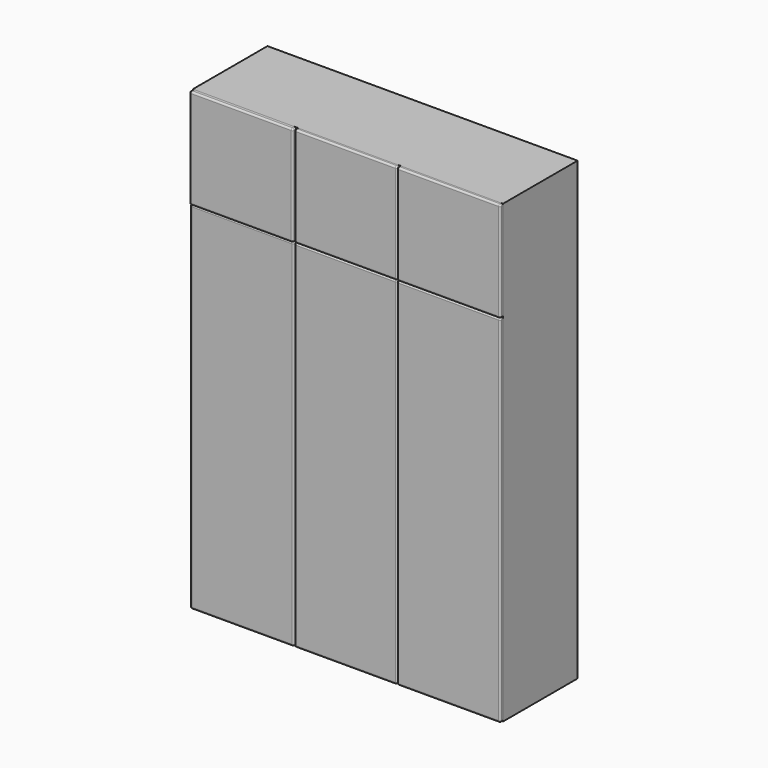
from build123d import *

# Parameters (mm, degrees)
F0_W      = 580
F0_H      = 280
F0_H_2    = 285
F0_H_3    = 175
F0_H_4    = 275
F0_H_5    = 560
F1_DEPTH  = 550
F0_W_2    = 590
F0_H_6    = 20
F5_W      = 610
F5_H      = 2100
F6_DEPTH  = 20
F7_R      = 10
F5_W_2    = 605
F8_DEPTH  = 20
F9_R      = 10
F10_DEPTH = 20
F11_R     = 10
F5_H_2    = 590
F12_DEPTH = 20
F13_R     = 10
F14_DEPTH = 20
F15_R     = 10
F16_DEPTH = 25
F17_R     = 10


# Not quite as in the source:
# - a feature names something its author has since deleted; it is built from what else it names
# - the program builds the solid bodies; features that only make, move or delete a surface that nothing else refers to are left out


with BuildPart() as f1:
    # F0 (on Front) → F1 (new body)
    with BuildSketch(Plane.XZ):
        Polygon((895, -1345), (915, -1345), (915, 1345), (-915, 1345), (-915, -1345), (-895, -1345), (-895, -755), (-315, -755), (-315, -1345), (-295, -1345), (-295, -395), (-295, -375), (-295, 625), (-295, 645), (-295, 745), (295, 745), (295, 645), (295, 625), (295, -375), (295, -395), (295, -1345), (315, -1345), (315, -1320), (315, -1140), (895, -1140), (895, -1320), align=None)
        with Locations((-605, -595)):
            Rectangle(F0_W, F0_H, mode=Mode.SUBTRACT)
        with Locations((-605, -292.5)):
            Rectangle(F0_W, F0_H_2, mode=Mode.SUBTRACT)
        with Locations((605, -1032.5)):
            Rectangle(F0_W, F0_H_3, mode=Mode.SUBTRACT)
        Polygon((315, 745), (895, 745), (895, 645), (895, 625), (895, -925), (315, -925), (315, 625), (315, 645), align=None, mode=Mode.SUBTRACT)
        with Locations((-605, 10)):
            Rectangle(F0_W, F0_H, mode=Mode.SUBTRACT)
        with Locations((-605, 310)):
            Rectangle(F0_W, F0_H, mode=Mode.SUBTRACT)
        with Locations((-605, 607.5)):
            Rectangle(F0_W, F0_H_4, mode=Mode.SUBTRACT)
        with Locations((-605, 1045)):
            Rectangle(F0_W, F0_H_5, mode=Mode.SUBTRACT)
        Polygon((-295, 1325), (895, 1325), (895, 765), (315, 765), (295, 765), (-295, 765), align=None, mode=Mode.SUBTRACT)
    extrude(amount=-F1_DEPTH)


with BuildPart() as f2:
    # F0 (on Front) → F2 (revolve)
    with BuildSketch(Plane.XZ):
        with Locations((0, 635)):
            Rectangle(F0_W_2, F0_H_6)
    revolve(axis=Axis((0, 0, 625), (-1, 0, 0)))


with BuildPart() as f2b:
    # F0 (on Front) → F2, piece 2 (revolve)
    with BuildSketch(Plane.XZ):
        with Locations((605, 635)):
            Rectangle(F0_W, F0_H_6)
    revolve(axis=Axis((0, 0, 625), (-1, 0, 0)))


with BuildPart() as f2_1:
    # F4: moved
    add(f2.part.moved(Location((0, 250, 0))))


with BuildPart() as f2b_1:
    # F4: moved
    add(f2b.part.moved(Location((0, 250, 0))))


with BuildPart() as f6:
    # F5 (on Front) → F6 (new body)
    with BuildSketch(Plane.XZ):
        with Locations((-610, -295)):
            Rectangle(F5_W, F5_H)
    extrude(amount=F6_DEPTH)

    # F7
    f7_edges = [f6.edges().sort_by_distance(p)[0] for p in [
        (-305, -10, 755),
        (-915, -10, 755),
        (-915, -10, -1345),
        (-305, -10, -1345),
        (-610, -20, -1345),
        (-305, -20, -295),
        (-610, -20, 755),
        (-915, -20, -295),
    ]]
    fillet(f7_edges, radius=F7_R)


with BuildPart() as f8:
    # F5 (on Front) → F8 (new body)
    with BuildSketch(Plane.XZ):
        with Locations((2.5, -295)):
            Rectangle(F5_W_2, F5_H)
    extrude(amount=F8_DEPTH)

    # F9
    f9_edges = [f8.edges().sort_by_distance(p)[0] for p in [
        (2.5, -20, -1345),
        (305, -20, -295),
        (2.5, -20, 755),
        (-300, -20, -295),
        (305, -10, 755),
        (-300, -10, 755),
        (305, -10, -1345),
        (-300, -10, -1345),
    ]]
    fillet(f9_edges, radius=F9_R)


with BuildPart() as f10:
    # F5 (on Front) → F10 (new body)
    with BuildSketch(Plane.XZ):
        with Locations((610, -295)):
            Rectangle(F5_W, F5_H)
    extrude(amount=F10_DEPTH)

    # F11
    f11_edges = [f10.edges().sort_by_distance(p)[0] for p in [
        (610, -20, -1345),
        (915, -20, -295),
        (610, -20, 755),
        (305, -20, -295),
        (915, -10, 755),
        (305, -10, 755),
        (305, -10, -1345),
        (915, -10, -1345),
    ]]
    fillet(f11_edges, radius=F11_R)


with BuildPart() as f12:
    # F5 (on Front) → F12 (new body)
    with BuildSketch(Plane.XZ):
        with Locations((610, 1050)):
            Rectangle(F5_W, F5_H_2)
    extrude(amount=F12_DEPTH)

    # F13
    f13_edges = [f12.edges().sort_by_distance(p)[0] for p in [
        (610, -20, 755),
        (915, -20, 1050),
        (610, -20, 1345),
        (305, -20, 1050),
        (915, -10, 1345),
        (915, -10, 755),
        (305, -10, 1345),
        (305, -10, 755),
    ]]
    fillet(f13_edges, radius=F13_R)


with BuildPart() as f14:
    # F5 (on Front) → F14 (new body)
    with BuildSketch(Plane.XZ):
        with Locations((2.5, 1050)):
            Rectangle(F5_W_2, F5_H_2)
    extrude(amount=F14_DEPTH)

    # F15
    f15_edges = [f14.edges().sort_by_distance(p)[0] for p in [
        (2.5, -20, 755),
        (305, -20, 1050),
        (2.5, -20, 1345),
        (-300, -20, 1050),
        (-300, -10, 1345),
        (305, -10, 1345),
        (305, -10, 755),
        (-300, -10, 755),
    ]]
    fillet(f15_edges, radius=F15_R)


with BuildPart() as f16:
    # F5 (on Front) → F16 (new body)
    with BuildSketch(Plane.XZ):
        with Locations((-610, 1050)):
            Rectangle(F5_W, F5_H_2)
    extrude(amount=F16_DEPTH)

    # F17
    f17_edges = [f16.edges().sort_by_distance(p)[0] for p in [
        (-610, -25, 755),
        (-305, -25, 1050),
        (-610, -25, 1345),
        (-915, -25, 1050),
        (-915, -12.5, 1345),
        (-305, -12.5, 1345),
        (-915, -12.5, 755),
        (-305, -12.5, 755),
    ]]
    fillet(f17_edges, radius=F17_R)


solid = Compound([f1.part, f2_1.part, f2b_1.part, f6.part, f8.part, f10.part, f12.part, f14.part, f16.part])
